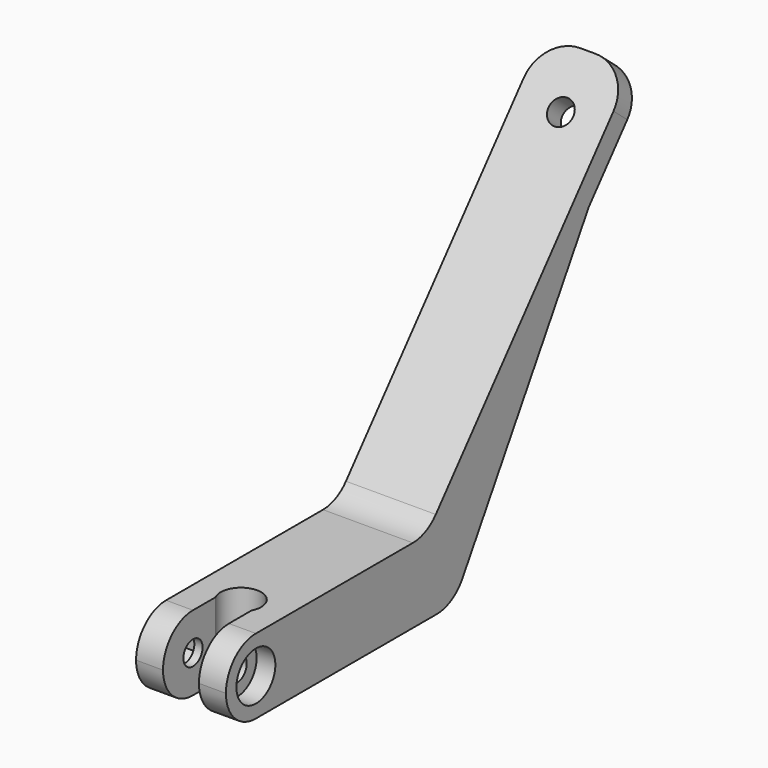
from build123d import *

# Parameters (mm, degrees)
F1_DEPTH  = 12
F3_DEPTH  = 25
F4_R      = 1.6
F5_DEPTH  = 12.001
F4_R_2    = 3.25
F6_DEPTH  = 2.5
F8_DEPTH  = 2.5
F9_R      = 1.65
F10_DEPTH = 34.5196429053
F11_R     = 4.99999


# Not quite as in the source:
# - a fillet or chamfer is up to 0.001 mm smaller than in the source, because OpenCascade refuses the exact size


with BuildPart() as f1:
    # F0 (on Right) → F1 (new body)
    with BuildSketch(Plane.YZ):
        Polygon((-19, 5), (-19, -5), (19, -5), (10.3397459622, 0), (14.535244118, 5), align=None)
        Polygon((10.3397459622, 0), (19, -5), (19, 5), (14.535244118, 5), align=None)
        Polygon((19, 5), (19, -5), (41.5633217274, 32.5436371113), (51.2051358727, 44.0343037581), (48.9070025433, 45.9626665871), (14.535244118, 5), align=None)
    extrude(amount=F1_DEPTH)

    # F2 (on face) → F3 (cut)
    with BuildSketch(Plane.XY.offset(5)):
        with BuildLine():
            ThreePointArc((8.4, -10.2369316877), (8.6239283527, -9.6363961031), (8.7, -9))
            ThreePointArc((8.7, -9), (5.3636038969, -6.3760716473), (3.6, -10.2369316877))
            Line((3.6, -10.2369316877), (8.4, -10.2369316877))
        make_face()
        with BuildLine():
            Line((8.4, -10.2369316877), (3.6, -10.2369316877))
            ThreePointArc((3.6, -10.2369316877), (6, -11.7), (8.4, -10.2369316877))
        make_face()
        with BuildLine():
            ThreePointArc((8.4, -10.2369316877), (6, -11.7), (3.6, -10.2369316877))
            Line((3.6, -10.2369316877), (3.6, -19))
            Line((3.6, -19), (8.4, -19))
            Line((8.4, -19), (8.4, -10.2369316877))
        make_face()
    extrude(amount=-F3_DEPTH, mode=Mode.SUBTRACT)

    # F4 (on face) → F5 (cut, through all)
    with BuildSketch(Plane.YZ.offset(12)):
        with Locations((-14, 0)):
            Circle(F4_R)
    extrude(amount=-F5_DEPTH, mode=Mode.SUBTRACT)

    # F4 (on face) → F6 (cut)
    with BuildSketch(Plane.YZ.offset(12)):
        with Locations((-14, 0)):
            Circle(F4_R_2)
        with Locations((-14, 0)):
            Circle(F4_R, mode=Mode.SUBTRACT)
    extrude(amount=-F6_DEPTH, mode=Mode.SUBTRACT)

    # F7 (on face) → F8 (cut)
    with BuildSketch(Plane(origin=(0, 0, 0), x_dir=(0, -1, 0), z_dir=(-1, 0, 0))):
        Polygon((11.15, 1.6454482672), (11.15, -1.6454482672), (14, -3.2908965344), (16.85, -1.6454482672), (16.85, 1.6454482672), (14, 3.2908965344), align=None)
    extrude(amount=-F8_DEPTH, mode=Mode.SUBTRACT)

    # F9 (on face) → F10 (cut, through all)
    with BuildSketch(Plane(origin=(0, 6.067612003, -5.0913309939), x_dir=(1, 0, 0), z_dir=(0, -0.7660444431, 0.6427876097))):
        with Locations((6, 59.6462605918)):
            Circle(F9_R)
    extrude(amount=-F10_DEPTH, mode=Mode.SUBTRACT)

    # F11 (radius 5 in the source; OpenCascade refuses exactly that, so slightly less here)
    f11_edges = [f1.edges().sort_by_distance(p)[0] for p in [
        (1.8, -19, 5),
        (10.2, -19, 5),
        (1.8, -19, -5),
        (10.2, -19, -5),
        (12, 50.056069, 44.998485),
        (0, 50.056069, 44.998485),
        (6, 14.535244, 5),
        (6, 19, -5),
    ]]
    fillet(f11_edges, radius=F11_R)


solid = f1.part
